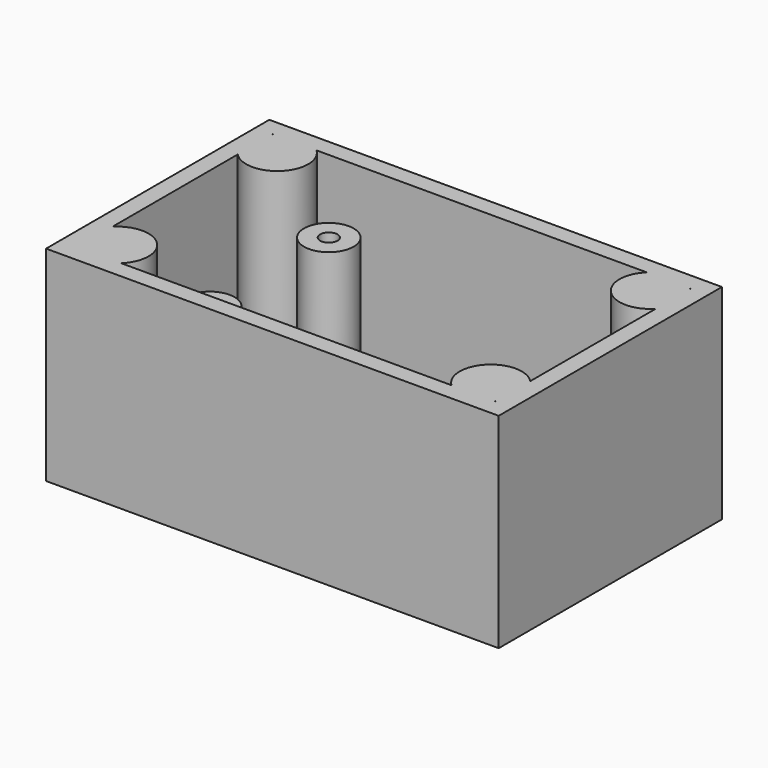
from build123d import *

# Parameters (mm, degrees)
F0_W             = 46.355
F0_H             = 28.575
F1_DEPTH         = 20.955
F2_T             = -1.778
F3_R             = 2.54
F4_DEPTH         = 14.986
F5_R             = 0.889
F6_DEPTH         = 6.35
F7_R             = 3.175
F8_DEPTH         = 19.177
F8_COPIES2_COUNT = 2


# Not quite as in the source:
# - a pattern or mirror of a feature is missing from the dataset's text; its kind, count and spacing are read off the source's solid


with BuildPart() as f1:
    # F0 (on Top) → F1 (new body)
    with BuildSketch(Plane.XY):
        Rectangle(F0_W, F0_H)
    extrude(amount=F1_DEPTH)

    # F2
    f2_openings = [f1.faces().sort_by_distance(p)[0] for p in [
        (0, 0, 20.955),
    ]]
    offset(amount=F2_T, openings=f2_openings)

    # F3 (on face) → F4 (join)
    with BuildSketch(Plane.XY.offset(1.778)):
        with Locations((-11.7475, -7.62)):
            Circle(F3_R)
    f4 = extrude(amount=F4_DEPTH)

    # F4_copies: F4 across plane
    add(f4.mirror(Plane.ZX))

    # F5 (on face) → F6 (cut)
    with BuildSketch(Plane.XY.offset(16.764)):
        with Locations((-11.7475, -7.62)):
            Circle(F5_R)
    f6 = extrude(amount=-F6_DEPTH, mode=Mode.SUBTRACT)

    # F6_copies: F6 across plane
    add(f6.mirror(Plane.ZX), mode=Mode.SUBTRACT)

    # F7 (on face) → F8 (join, through all)
    with BuildSketch(Plane.XY.offset(1.778)):
        with Locations((-19.1135, -10.2235)):
            Circle(F7_R)
    f8 = extrude(amount=F8_DEPTH)

    # F8_copies: F8 across plane
    add(f8.mirror(Plane.ZX))

    # F8_copies1: F8 across plane
    add(f8.mirror(Plane(origin=(0, 0, 0), x_dir=(0, 0, 1), z_dir=(1, 0, 0))))

    # F8_copies2: F8 ×2 about axis
    f8_copies2_axis = Axis((0, 0, 0), (0, 0, 1))
    for i in range(1, F8_COPIES2_COUNT):
        add(f8.rotate(f8_copies2_axis, i * 360 / F8_COPIES2_COUNT))


solid = f1.part
